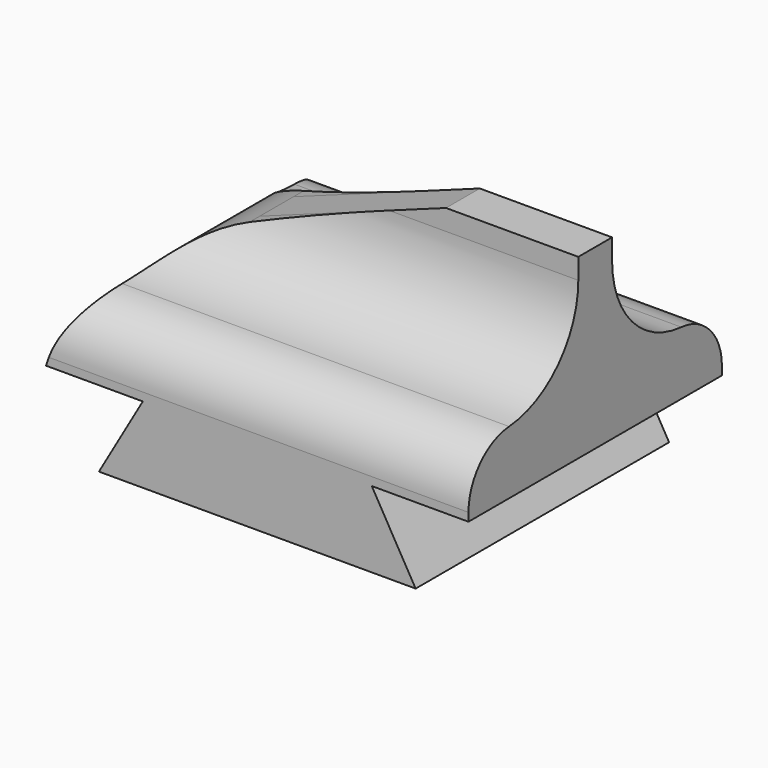
from build123d import *

# Parameters (mm, degrees)
F0_W         = 9.525
F0_H         = 9.525
F1_DEPTH     = 2.286
F2_T1_DEPTH  = 21.3619144247
F3_W         = 2.9083
F3_H         = 9.525
F3_W_2       = 6.8834
F4_DEPTH     = 1.905
F5_R         = 1.6556676611
F6_W         = 12.7
F6_H         = 1.27
F7_DEPTH     = 3.429
F8_SIZE2     = 8.7232408068
F8_SIZE      = 3.175
F9_T4_DEPTH  = 12.7
F9_T9_DEPTH  = 12.7
F10_T1_DEPTH = 21.1289299719


# Not quite as in the source:
# - a fillet or chamfer that OpenCascade refuses, or shapes differently, is made with other operations: its cross-section is extruded or revolved along the edge and cut away or added


with BuildPart() as f1:
    # F0 (on Top) → F1 (new body)
    with BuildSketch(Plane.XY):
        Rectangle(F0_W, F0_H)
    extrude(amount=F1_DEPTH)

    # F2: chamfer of 1.3208 x 2.2876927066 on 2 edges, made by hand

    # F2_s2 → F2_t1 (cut)
    with BuildSketch(Plane.XZ.offset(-10.6809572123)):
        Polygon((-4.7625, -0.0016927066), (-3.4417, 2.286), (-4.7625, 2.286), align=None)
        Polygon((4.7625, -0.0016927066), (3.4417, 2.286), (4.7625, 2.286), align=None)
    extrude(amount=F2_T1_DEPTH, mode=Mode.SUBTRACT)

    # F3 (on face) → F4 (join)
    with BuildSketch(Plane.XY.offset(2.286)):
        with Locations((4.89585, 0)):
            Rectangle(F3_W, F3_H)
        Rectangle(F3_W_2, F3_H)
        with Locations((-4.89585, 0)):
            Rectangle(F3_W, F3_H)
    extrude(amount=F4_DEPTH)

    # F5
    f5_edges = [f1.edges().sort_by_distance(p)[0] for p in [
        (0, 4.7625, 4.191),
        (0, -4.7625, 4.191),
    ]]
    fillet(f5_edges, radius=F5_R)

    # F6 (on face) → F7 (join)
    with BuildSketch(Plane.XY.offset(4.191)):
        Rectangle(F6_W, F6_H)
    extrude(amount=F7_DEPTH)

    # F8
    f8_edges = [f1.edges().sort_by_distance(p)[0] for p in [
        (-6.35, 0, 7.62),
    ]]
    f8_side = f1.faces().sort_by_distance((-6.35, 0, 3.751025))[0]
    chamfer(f8_edges, length=F8_SIZE, length2=F8_SIZE2, reference=f8_side)

    # F9: fillet of radius 2.8207671263 on 2 edges, made by hand


with BuildPart() as f9_tool2:
    # F9_s3 → F9_t4 (new body)
    with BuildSketch(Plane.YZ.offset(-6.35)):
        with BuildLine():
            ThreePointArc((-0.635, 6.9981468006), (-1.3849039981, 5.0828783899), (-3.235890411, 4.1859623453))
            Line((-3.235890411, 4.1859623453), (-3.2139027394, 3.9047438998))
            ThreePointArc((-3.2139027394, 3.9047438998), (-3.1068323389, 3.9089232874), (-0.635, 3.9089232874))
            Line((-0.635, 3.9089232874), (-0.3529232874, 4.191))
            Line((-0.3529232874, 4.191), (-0.3529232874, 6.9981468006))
            Line((-0.3529232874, 6.9981468006), (-0.635, 6.9981468006))
        make_face()
    extrude(amount=F9_T4_DEPTH)

    split(bisect_by=Plane(origin=(-2.1714043556, 0, 5.9658844356), x_dir=(0, 1, 0), z_dir=(0.3420201433, 0, -0.9396926208)), keep=Keep.TOP)


with BuildPart() as f1_1:
    add(f1.part)

    # F9_t1: union F9_tool2
    add(f9_tool2.part)


with BuildPart() as f9_tool7:
    # F9_s8 → F9_t9 (new body)
    with BuildSketch(Plane.YZ.offset(6.35)):
        with BuildLine():
            ThreePointArc((0.635, 6.9981468006), (1.3849039981, 5.0828783899), (3.235890411, 4.1859623453))
            Line((3.235890411, 4.1859623453), (3.2139027394, 3.9047438998))
            ThreePointArc((3.2139027394, 3.9047438998), (3.1068323389, 3.9089232874), (0.635, 3.9089232874))
            Line((0.635, 3.9089232874), (0.3529232874, 4.191))
            Line((0.3529232874, 4.191), (0.3529232874, 6.9981468006))
            Line((0.3529232874, 6.9981468006), (0.635, 6.9981468006))
        make_face()
    extrude(amount=-F9_T9_DEPTH)

    split(bisect_by=Plane(origin=(-2.1714043556, 0, 5.9658844356), x_dir=(0, 1, 0), z_dir=(0.3420201433, 0, -0.9396926208)), keep=Keep.TOP)


with BuildPart() as f1_2:
    add(f1_1.part)

    # F9_t6: union F9_tool7
    add(f9_tool7.part)

    # F10: fillet of radius 5.08 on 1 edges, made by hand

    # F10_s2 → F10_t1 (cut)
    with BuildSketch(Plane.XZ.offset(-10.564464986)):
        with BuildLine():
            ThreePointArc((-6.35, 2.286), (-5.1772680397, 4.3020632997), (-3.2272380907, 5.5815923837))
            Line((-3.2272380907, 5.5815923837), (-3.2619873372, 5.677065154))
            Line((-3.2619873372, 5.677065154), (-6.3847492466, 4.5404727703))
            Line((-6.3847492466, 4.5404727703), (-6.4516, 4.445))
            ThreePointArc((-6.4516, 4.445), (-6.4516, 3.3655), (-6.4472044847, 2.3155609226))
            Line((-6.4472044847, 2.3155609226), (-6.35, 2.286))
        make_face()
    extrude(amount=F10_T1_DEPTH, mode=Mode.SUBTRACT)


solid = f1_2.part
